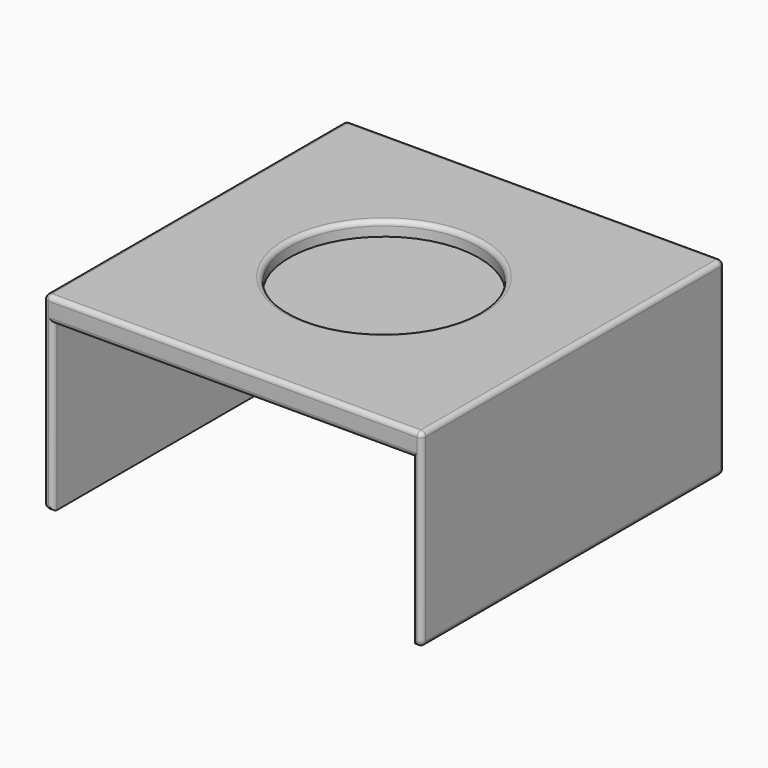
from build123d import *

# Parameters (mm, degrees)
F0_W          = 80
F0_H          = 40
F1_DEPTH      = 40
F1_DEPTH_BACK = 40
F2_W          = 76
F2_H          = 35
F3_DEPTH      = 78
F4_R          = 20.05
F5_DEPTH      = 3
F6_R          = 0.99999


# Not quite as in the source:
# - a fillet or chamfer is up to 0.001 mm smaller than in the source, because OpenCascade refuses the exact size


with BuildPart() as f1:
    # F0 (on Front) → F1 (new body, two sides)
    with BuildSketch(Plane.XZ) as f1_sk:
        Rectangle(F0_W, F0_H)
    extrude(amount=F1_DEPTH)
    extrude(f1_sk.sketch, amount=-F1_DEPTH_BACK)

    # F2 (on face) → F3 (cut)
    with BuildSketch(Plane.XZ.offset(40)):
        with Locations((0, -2.5)):
            Rectangle(F2_W, F2_H)
    extrude(amount=-F3_DEPTH, mode=Mode.SUBTRACT)

    # F4 (on face) → F5 (cut)
    with BuildSketch(Plane.XY.offset(20)):
        Circle(F4_R)
    extrude(amount=-F5_DEPTH, mode=Mode.SUBTRACT)

    # F6 (radius 1 in the source; OpenCascade refuses exactly that, so slightly less here)
    f6_edges = [f1.edges().sort_by_distance(p)[0] for p in [
        (40, -40, 0),
        (40, 0, 20),
        (40, 40, 0),
        (40, 0, -20),
        (-40, -40, 0),
        (0, -40, 20),
        (39, -40, -20),
        (38, -40, -2.5),
        (0, -40, 15),
        (-38, -40, -2.5),
        (-39, -40, -20),
        (-40, 0, 20),
        (0, 40, 20),
        (-20.05, 0, 20),
        (0, 40, -20),
        (-40, 40, 0),
        (-40, 0, -20),
    ]]
    fillet(f6_edges, radius=F6_R)


solid = f1.part
